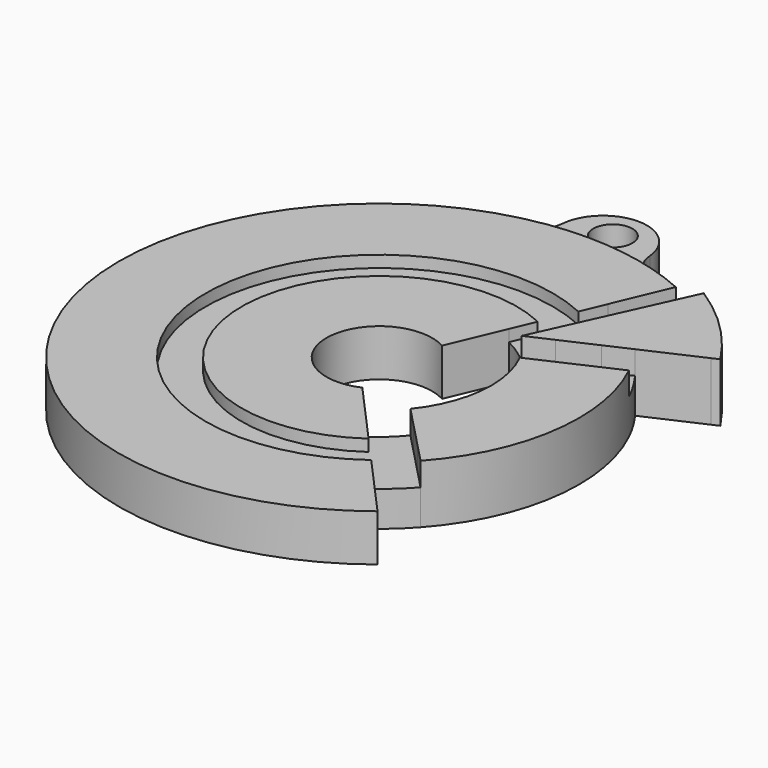
from build123d import *

# Parameters (mm, degrees)
F0_R        = 1.5044645314
F1_DEPTH    = 2.7
F2_DEPTH    = 0.9
F3_DEPTH    = 2.7
F4_DEPTH    = 1.8
F5_T1_DEPTH = 2.7


# Not quite as in the source:
# - a fillet or chamfer that OpenCascade refuses, or shapes differently, is made with other operations: its cross-section is extruded or revolved along the edge and cut away or added


with BuildPart() as f1:
    # F0 (on Top) → F1 (new body)
    with BuildSketch(Plane.XY):
        with BuildLine():
            ThreePointArc((-2.9059050305, 19.7877668258), (-18.361479671, -7.928181651), (12.4102011034, -15.6839697964))
            Line((12.4102011034, -15.6839697964), (9.3065271924, -12.2254227754))
            ThreePointArc((9.3065271924, -12.2254227754), (-15.2699304913, -1.7034180964), (6.3836906961, 13.9757255095))
            Line((6.3836906961, 13.9757255095), (8.1864677167, 18.2477874364))
            ThreePointArc((8.1864677167, 18.2477874364), (5.5993809855, 19.2001805351), (2.9059050305, 19.7877668258))
            ThreePointArc((2.9059050305, 19.7877668258), (0, 18.1241204417), (-2.9059050305, 19.7877668258))
        make_face()
        with BuildLine():
            ThreePointArc((6.3836906961, 13.9757255095), (-15.2699304913, -1.7034180964), (9.3065271924, -12.2254227754))
            Line((9.3065271924, -12.2254227754), (7.9527661976, -10.7168731694))
            ThreePointArc((7.9527661976, -10.7168731694), (-13.2749249311, -1.3690247612), (5.5982117915, 12.114366903))
            Line((5.5982117915, 12.114366903), (6.3836906961, 13.9757255095))
        make_face()
        with BuildLine():
            ThreePointArc((5.5982117915, 12.114366903), (-13.2749249311, -1.3690247612), (7.9527661976, -10.7168731694))
            Line((7.9527661976, -10.7168731694), (6.0964799797, -8.6483397626))
            ThreePointArc((6.0964799797, -8.6483397626), (-10.5418803683, -0.9108276969), (4.5227579261, 9.5658512185))
            Line((4.5227579261, 9.5658512185), (5.5982117915, 12.114366903))
        make_face()
        with BuildLine():
            ThreePointArc((4.5227579261, 9.5658512185), (-10.5418803683, -0.9108276969), (6.0964799797, -8.6483397626))
            Line((6.0964799797, -8.6483397626), (4.7718042528, -7.1722010249))
            ThreePointArc((4.7718042528, -7.1722010249), (-8.5947223482, -0.5842355063), (3.7573171653, 7.7519772374))
            Line((3.7573171653, 7.7519772374), (4.5227579261, 9.5658512185))
        make_face()
        with BuildLine():
            ThreePointArc((3.7573171653, 7.7519772374), (-8.5947223482, -0.5842355063), (4.7718042528, -7.1722010249))
            Line((4.7718042528, -7.1722010249), (1.6593857385, -3.7039095455))
            ThreePointArc((1.6593857385, -3.7039095455), (-4.0546444127, 0.1799045205), (1.9809039535, 3.5423899386))
            Line((1.9809039535, 3.5423899386), (3.7573171653, 7.7519772374))
        make_face()
        with BuildLine():
            ThreePointArc((2.9059050305, 19.7877668258), (0, 20), (-2.9059050305, 19.7877668258))
            ThreePointArc((-2.9059050305, 19.7877668258), (0, 18.1241204417), (2.9059050305, 19.7877668258))
        make_face()
        with BuildLine():
            ThreePointArc((-3.157685128, 20.3174125427), (-3.043339046, 20.0471019762), (-2.9059050305, 19.7877668258))
            ThreePointArc((-2.9059050305, 19.7877668258), (0, 20), (2.9059050305, 19.7877668258))
            ThreePointArc((2.9059050305, 19.7877668258), (3.043339046, 20.0471019762), (3.157685128, 20.3174125427))
            ThreePointArc((3.157685128, 20.3174125427), (0, 20.5613284541), (-3.157685128, 20.3174125427))
        make_face()
        with BuildLine():
            ThreePointArc((3.3697074825, 21.4938279241), (-0.5976844127, 24.8101062388), (-3.157685128, 20.3174125427))
            ThreePointArc((-3.157685128, 20.3174125427), (0, 20.5613284541), (3.157685128, 20.3174125427))
            ThreePointArc((3.157685128, 20.3174125427), (3.3162783146, 20.8961435115), (3.3697074825, 21.4938279241))
        make_face()
        with Locations((0, 22.4330537021)):
            Circle(F0_R, mode=Mode.SUBTRACT)
        with BuildLine():
            ThreePointArc((13.8344540426, 6.6843318112), (13.1730545976, 7.9084159596), (12.4036340143, 9.0676498421))
            Line((12.4036340143, 9.0676498421), (10.5172175152, 8.21498609))
            ThreePointArc((10.5172175152, 8.21498609), (11.318131065, 7.0709101194), (11.995098321, 5.8493997121))
            Line((11.995098321, 5.8493997121), (13.8344540426, 6.6843318112))
        make_face()
        with BuildLine():
            ThreePointArc((11.995098321, 5.8493997121), (11.318131065, 7.0709101194), (10.5172175152, 8.21498609))
            Line((10.5172175152, 8.21498609), (7.9045951482, 7.0340759404))
            ThreePointArc((7.9045951482, 7.0340759404), (8.7683299388, 5.9226040621), (9.4768887451, 4.706317935))
            Line((9.4768887451, 4.706317935), (11.995098321, 5.8493997121))
        make_face()
        with BuildLine():
            ThreePointArc((9.4768887451, 4.706317935), (8.7683299388, 5.9226040621), (7.9045951482, 7.0340759404))
            Line((7.9045951482, 7.0340759404), (6.0058132946, 6.1758230253))
            ThreePointArc((6.0058132946, 6.1758230253), (6.9398340598, 5.1038501734), (7.6848114732, 3.8928467719))
            Line((7.6848114732, 3.8928467719), (9.4768887451, 4.706317935))
        make_face()
        with BuildLine():
            Line((6.0058132946, 6.1758230253), (7.9045951482, 7.0340759404))
            ThreePointArc((7.9045951482, 7.0340759404), (7.4001814409, 7.5629467428), (6.8604632985, 8.0557365971))
            Line((6.8604632985, 8.0557365971), (6.0058132946, 6.1758230253))
        make_face()
        with BuildLine():
            ThreePointArc((6.8604632985, 8.0557365971), (5.7414756731, 8.8879866049), (4.5227579261, 9.5658512185))
            Line((4.5227579261, 9.5658512185), (3.7573171653, 7.7519772374))
            ThreePointArc((3.7573171653, 7.7519772374), (4.9447694202, 7.0540654058), (6.0058132946, 6.1758230253))
            Line((6.0058132946, 6.1758230253), (6.8604632985, 8.0557365971))
        make_face()
        with BuildLine():
            ThreePointArc((8.0404414582, 10.6512516579), (6.8584540657, 11.4481207432), (5.5982117915, 12.114366903))
            Line((5.5982117915, 12.114366903), (4.5227579261, 9.5658512185))
            ThreePointArc((4.5227579261, 9.5658512185), (5.7414756731, 8.8879866049), (6.8604632985, 8.0557365971))
            Line((6.8604632985, 8.0557365971), (8.0404414582, 10.6512516579))
        make_face()
        with BuildLine():
            ThreePointArc((8.8939895289, 12.5287413845), (7.6730254156, 13.3115397829), (6.3836906961, 13.9757255095))
            Line((6.3836906961, 13.9757255095), (5.5982117915, 12.114366903))
            ThreePointArc((5.5982117915, 12.114366903), (6.8584540657, 11.4481207432), (8.0404414582, 10.6512516579))
            Line((8.0404414582, 10.6512516579), (8.8939895289, 12.5287413845))
        make_face()
        with BuildLine():
            Line((7.9045951482, 7.0340759404), (10.5172175152, 8.21498609))
            ThreePointArc((10.5172175152, 8.21498609), (9.3584466725, 9.514059943), (8.0404414582, 10.6512516579))
            Line((8.0404414582, 10.6512516579), (6.8604632985, 8.0557365971))
            ThreePointArc((6.8604632985, 8.0557365971), (7.4001814409, 7.5629467428), (7.9045951482, 7.0340759404))
        make_face()
        with BuildLine():
            Line((10.5172175152, 8.21498609), (12.4036340143, 9.0676498421))
            ThreePointArc((12.4036340143, 9.0676498421), (10.7885115198, 10.9398550999), (8.8939895289, 12.5287413845))
            Line((8.8939895289, 12.5287413845), (8.0404414582, 10.6512516579))
            ThreePointArc((8.0404414582, 10.6512516579), (9.3584466725, 9.514059943), (10.5172175152, 8.21498609))
        make_face()
        with BuildLine():
            Line((12.4036340143, 9.0676498421), (16.6976556484, 11.008555575))
            ThreePointArc((16.6976556484, 11.008555575), (14.070563524, 14.2133473227), (10.8394114429, 16.807949297))
            Line((10.8394114429, 16.807949297), (8.8939895289, 12.5287413845))
            ThreePointArc((8.8939895289, 12.5287413845), (10.7885115198, 10.9398550999), (12.4036340143, 9.0676498421))
        make_face()
        with BuildLine():
            ThreePointArc((10.8394114429, 16.807949297), (14.070563524, 14.2133473227), (16.6976556484, 11.008555575))
            Line((16.6976556484, 11.008555575), (17.2154603994, 11.2426042817))
            ThreePointArc((17.2154603994, 11.2426042817), (14.4679762691, 14.6097874889), (11.0741551061, 17.3242984413))
            Line((11.0741551061, 17.3242984413), (10.8394114429, 16.807949297))
        make_face()
    extrude(amount=-F1_DEPTH)

    # F0 (on Top) → F2 (join)
    with BuildSketch(Plane.XY):
        with BuildLine():
            ThreePointArc((-2.9059050305, 19.7877668258), (-18.361479671, -7.928181651), (12.4102011034, -15.6839697964))
            Line((12.4102011034, -15.6839697964), (9.3065271924, -12.2254227754))
            ThreePointArc((9.3065271924, -12.2254227754), (-15.2699304913, -1.7034180964), (6.3836906961, 13.9757255095))
            Line((6.3836906961, 13.9757255095), (8.1864677167, 18.2477874364))
            ThreePointArc((8.1864677167, 18.2477874364), (5.5993809855, 19.2001805351), (2.9059050305, 19.7877668258))
            ThreePointArc((2.9059050305, 19.7877668258), (0, 18.1241204417), (-2.9059050305, 19.7877668258))
        make_face()
        with BuildLine():
            ThreePointArc((6.3836906961, 13.9757255095), (-15.2699304913, -1.7034180964), (9.3065271924, -12.2254227754))
            Line((9.3065271924, -12.2254227754), (7.9527661976, -10.7168731694))
            ThreePointArc((7.9527661976, -10.7168731694), (-13.2749249311, -1.3690247612), (5.5982117915, 12.114366903))
            Line((5.5982117915, 12.114366903), (6.3836906961, 13.9757255095))
        make_face()
        with BuildLine():
            ThreePointArc((4.5227579261, 9.5658512185), (-10.5418803683, -0.9108276969), (6.0964799797, -8.6483397626))
            Line((6.0964799797, -8.6483397626), (4.7718042528, -7.1722010249))
            ThreePointArc((4.7718042528, -7.1722010249), (-8.5947223482, -0.5842355063), (3.7573171653, 7.7519772374))
            Line((3.7573171653, 7.7519772374), (4.5227579261, 9.5658512185))
        make_face()
        with BuildLine():
            ThreePointArc((3.7573171653, 7.7519772374), (-8.5947223482, -0.5842355063), (4.7718042528, -7.1722010249))
            Line((4.7718042528, -7.1722010249), (1.6593857385, -3.7039095455))
            ThreePointArc((1.6593857385, -3.7039095455), (-4.0546444127, 0.1799045205), (1.9809039535, 3.5423899386))
            Line((1.9809039535, 3.5423899386), (3.7573171653, 7.7519772374))
        make_face()
        with BuildLine():
            ThreePointArc((2.9059050305, 19.7877668258), (0, 20), (-2.9059050305, 19.7877668258))
            ThreePointArc((-2.9059050305, 19.7877668258), (0, 18.1241204417), (2.9059050305, 19.7877668258))
        make_face()
    extrude(amount=F2_DEPTH)

    # F0 (on Top) → F3 (join)
    with BuildSketch(Plane.XY):
        with BuildLine():
            Line((6.7113864418, -5.4007291543), (8.0821585416, -6.8293163715))
            ThreePointArc((8.0821585416, -6.8293163715), (9.9367857977, -3.6360881181), (10.5811553619, 0))
            ThreePointArc((10.5811553619, 0), (10.3013902205, 2.4170660555), (9.4768887451, 4.706317935))
            Line((9.4768887451, 4.706317935), (7.6848114732, 3.8928467719))
            ThreePointArc((7.6848114732, 3.8928467719), (8.3788968801, 2.00116727), (8.6145564813, 0))
            ThreePointArc((8.6145564813, 0), (8.1248446428, -2.8631246741), (6.7113864418, -5.4007291543))
        make_face()
        with BuildLine():
            Line((8.0821585416, -6.8293163715), (10.0042554899, -8.8324816906))
            ThreePointArc((10.0042554899, -8.8324816906), (12.4821464921, -4.721639511), (13.3453310458, 0))
            ThreePointArc((13.3453310458, 0), (13.0033922255, 3.0016081275), (11.995098321, 5.8493997121))
            Line((11.995098321, 5.8493997121), (9.4768887451, 4.706317935))
            ThreePointArc((9.4768887451, 4.706317935), (10.3013902205, 2.4170660555), (10.5811553619, 0))
            ThreePointArc((10.5811553619, 0), (9.9367857977, -3.6360881181), (8.0821585416, -6.8293163715))
        make_face()
        with BuildLine():
            Line((10.0042554899, -8.8324816906), (11.4065098197, -10.2938789654))
            ThreePointArc((11.4065098197, -10.2938789654), (14.3410149492, -5.5143177862), (15.3646480734, 0))
            ThreePointArc((15.3646480734, 0), (14.9772148291, 3.4286216448), (13.8344540426, 6.6843318112))
            Line((13.8344540426, 6.6843318112), (11.995098321, 5.8493997121))
            ThreePointArc((11.995098321, 5.8493997121), (13.0033922255, 3.0016081275), (13.3453310458, 0))
            ThreePointArc((13.3453310458, 0), (12.4821464921, -4.721639511), (10.0042554899, -8.8324816906))
        make_face()
        with BuildLine():
            Line((7.9527661976, -10.7168731694), (9.3065271924, -12.2254227754))
            ThreePointArc((9.3065271924, -12.2254227754), (10.4014513861, -11.3085020883), (11.4065098197, -10.2938789654))
            Line((11.4065098197, -10.2938789654), (10.0042554899, -8.8324816906))
            ThreePointArc((10.0042554899, -8.8324816906), (9.0278120152, -9.8283503672), (7.9527661976, -10.7168731694))
        make_face()
        with BuildLine():
            Line((6.0964799797, -8.6483397626), (7.9527661976, -10.7168731694))
            ThreePointArc((7.9527661976, -10.7168731694), (9.0278120152, -9.8283503672), (10.0042554899, -8.8324816906))
            Line((10.0042554899, -8.8324816906), (8.0821585416, -6.8293163715))
            ThreePointArc((8.0821585416, -6.8293163715), (7.1474232492, -7.8022554232), (6.0964799797, -8.6483397626))
        make_face()
        with BuildLine():
            Line((4.7718042528, -7.1722010249), (6.0964799797, -8.6483397626))
            ThreePointArc((6.0964799797, -8.6483397626), (7.1474232492, -7.8022554232), (8.0821585416, -6.8293163715))
            Line((8.0821585416, -6.8293163715), (6.7113864418, -5.4007291543))
            ThreePointArc((6.7113864418, -5.4007291543), (5.8095133427, -6.3608284122), (4.7718042528, -7.1722010249))
        make_face()
    extrude(amount=-F3_DEPTH)

    # F0 (on Top) → F4 (join)
    with BuildSketch(Plane.XY):
        with BuildLine():
            Line((10.0042554899, -8.8324816906), (11.4065098197, -10.2938789654))
            ThreePointArc((11.4065098197, -10.2938789654), (14.3410149492, -5.5143177862), (15.3646480734, 0))
            ThreePointArc((15.3646480734, 0), (14.9772148291, 3.4286216448), (13.8344540426, 6.6843318112))
            Line((13.8344540426, 6.6843318112), (11.995098321, 5.8493997121))
            ThreePointArc((11.995098321, 5.8493997121), (13.0033922255, 3.0016081275), (13.3453310458, 0))
            ThreePointArc((13.3453310458, 0), (12.4821464921, -4.721639511), (10.0042554899, -8.8324816906))
        make_face()
        with BuildLine():
            Line((8.0821585416, -6.8293163715), (10.0042554899, -8.8324816906))
            ThreePointArc((10.0042554899, -8.8324816906), (12.4821464921, -4.721639511), (13.3453310458, 0))
            ThreePointArc((13.3453310458, 0), (13.0033922255, 3.0016081275), (11.995098321, 5.8493997121))
            Line((11.995098321, 5.8493997121), (9.4768887451, 4.706317935))
            ThreePointArc((9.4768887451, 4.706317935), (10.3013902205, 2.4170660555), (10.5811553619, 0))
            ThreePointArc((10.5811553619, 0), (9.9367857977, -3.6360881181), (8.0821585416, -6.8293163715))
        make_face()
        with BuildLine():
            Line((6.7113864418, -5.4007291543), (8.0821585416, -6.8293163715))
            ThreePointArc((8.0821585416, -6.8293163715), (9.9367857977, -3.6360881181), (10.5811553619, 0))
            ThreePointArc((10.5811553619, 0), (10.3013902205, 2.4170660555), (9.4768887451, 4.706317935))
            Line((9.4768887451, 4.706317935), (7.6848114732, 3.8928467719))
            ThreePointArc((7.6848114732, 3.8928467719), (8.3788968801, 2.00116727), (8.6145564813, 0))
            ThreePointArc((8.6145564813, 0), (8.1248446428, -2.8631246741), (6.7113864418, -5.4007291543))
        make_face()
        with BuildLine():
            ThreePointArc((10.8394114429, 16.807949297), (14.070563524, 14.2133473227), (16.6976556484, 11.008555575))
            Line((16.6976556484, 11.008555575), (17.2154603994, 11.2426042817))
            ThreePointArc((17.2154603994, 11.2426042817), (14.4679762691, 14.6097874889), (11.0741551061, 17.3242984413))
            Line((11.0741551061, 17.3242984413), (10.8394114429, 16.807949297))
        make_face()
        with BuildLine():
            Line((6.0058132946, 6.1758230253), (7.9045951482, 7.0340759404))
            ThreePointArc((7.9045951482, 7.0340759404), (7.4001814409, 7.5629467428), (6.8604632985, 8.0557365971))
            Line((6.8604632985, 8.0557365971), (6.0058132946, 6.1758230253))
        make_face()
        with BuildLine():
            Line((7.9045951482, 7.0340759404), (10.5172175152, 8.21498609))
            ThreePointArc((10.5172175152, 8.21498609), (9.3584466725, 9.514059943), (8.0404414582, 10.6512516579))
            Line((8.0404414582, 10.6512516579), (6.8604632985, 8.0557365971))
            ThreePointArc((6.8604632985, 8.0557365971), (7.4001814409, 7.5629467428), (7.9045951482, 7.0340759404))
        make_face()
        with BuildLine():
            Line((10.5172175152, 8.21498609), (12.4036340143, 9.0676498421))
            ThreePointArc((12.4036340143, 9.0676498421), (10.7885115198, 10.9398550999), (8.8939895289, 12.5287413845))
            Line((8.8939895289, 12.5287413845), (8.0404414582, 10.6512516579))
            ThreePointArc((8.0404414582, 10.6512516579), (9.3584466725, 9.514059943), (10.5172175152, 8.21498609))
        make_face()
        with BuildLine():
            Line((12.4036340143, 9.0676498421), (16.6976556484, 11.008555575))
            ThreePointArc((16.6976556484, 11.008555575), (14.070563524, 14.2133473227), (10.8394114429, 16.807949297))
            Line((10.8394114429, 16.807949297), (8.8939895289, 12.5287413845))
            ThreePointArc((8.8939895289, 12.5287413845), (10.7885115198, 10.9398550999), (12.4036340143, 9.0676498421))
        make_face()
    extrude(amount=F4_DEPTH)

    # F5: fillet of radius 3 on 2 edges, made by hand

    # F5_s2 → F5_t1 (join)
    with BuildSketch(Plane.XY.offset(-2.7)):
        with BuildLine():
            ThreePointArc((3.3539587166, 21.8192345075), (4.0340965589, 20.1897997022), (5.5129894146, 19.2251644392))
            ThreePointArc((5.5129894146, 19.2251644392), (4.2188358916, 19.5499724736), (2.9059050305, 19.7877668258))
            ThreePointArc((2.9059050305, 19.7877668258), (3.2906213347, 20.768059539), (3.3539587166, 21.8192345075))
        make_face()
        with BuildLine():
            ThreePointArc((-3.3539587166, 21.8192345075), (-4.0340965589, 20.1897997022), (-5.5129894146, 19.2251644392))
            ThreePointArc((-5.5129894146, 19.2251644392), (-4.2188358916, 19.5499724736), (-2.9059050305, 19.7877668258))
            ThreePointArc((-2.9059050305, 19.7877668258), (-3.2906213347, 20.768059539), (-3.3539587166, 21.8192345075))
        make_face()
    extrude(amount=F5_T1_DEPTH)


solid = f1.part
